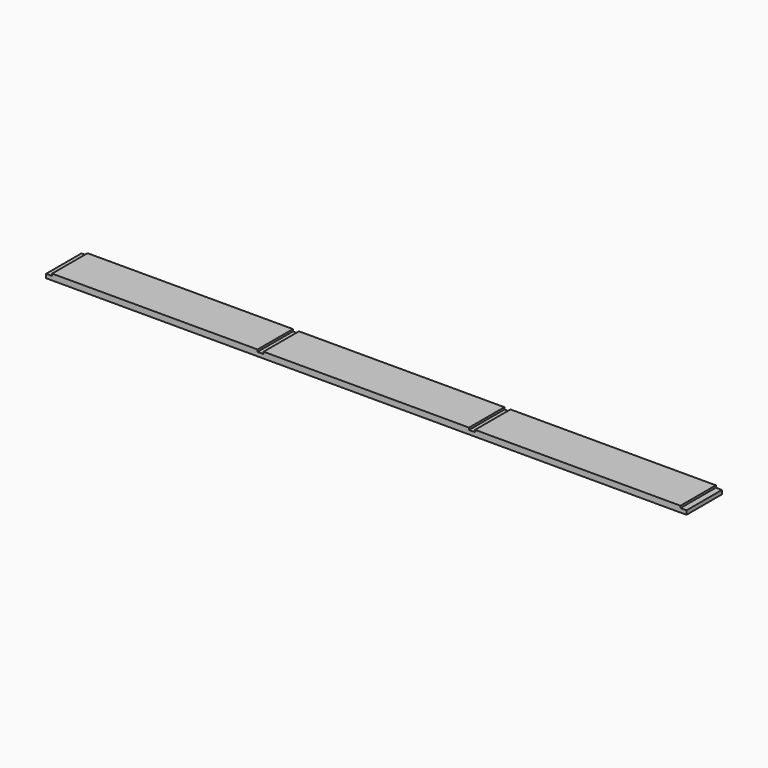
from build123d import *

# Parameters (mm, degrees)
F0_W     = 1930.4
F0_H     = 133.35
F1_DEPTH = 18.25625
F2_W     = 18.25625
F2_H     = 6.35
F3_DEPTH = 133.351
F4_W     = 18.25625
F4_H     = 6.35
F5_DEPTH = 133.351
F6_W     = 18.25625
F6_H     = 6.35
F7_DEPTH = 133.351
F8_W     = 18.25625
F8_H     = 6.35
F9_DEPTH = 133.351


# Not quite as in the source:
# - a length typed as a fraction of an inch, garbled in the dataset ("3 / 203.2 mm" for 3/8 in), is restored


with BuildPart() as f1:
    # F0 (on Top) → F1 (new body)
    with BuildSketch(Plane.XY):
        with Locations((302.4911884634, -268.7286456764)):
            Rectangle(F0_W, F0_H)
    extrude(amount=-F1_DEPTH)

    # F2 (on face) → F3 (cut, through all)
    with BuildSketch(Plane.XZ.offset(335.4036456764)):
        with Locations((-653.5806865366, -3.175)):
            Rectangle(F2_W, F2_H)
    extrude(amount=-F3_DEPTH, mode=Mode.SUBTRACT)

    # F4 (on face) → F5 (cut, through all)
    with BuildSketch(Plane.XZ.offset(335.4036456764)):
        with Locations((1258.5630634634, -3.175)):
            Rectangle(F4_W, F4_H)
    extrude(amount=-F5_DEPTH, mode=Mode.SUBTRACT)

    # F6 (on face) → F7 (cut, through all)
    with BuildSketch(Plane.XZ.offset(335.4036456764)):
        with Locations((621.1818134634, -3.175)):
            Rectangle(F6_W, F6_H)
    extrude(amount=-F7_DEPTH, mode=Mode.SUBTRACT)

    # F8 (on face) → F9 (cut, through all)
    with BuildSketch(Plane.XZ.offset(335.4036456764)):
        with Locations((-16.1994365366, -3.175)):
            Rectangle(F8_W, F8_H)
    extrude(amount=-F9_DEPTH, mode=Mode.SUBTRACT)


solid = f1.part
